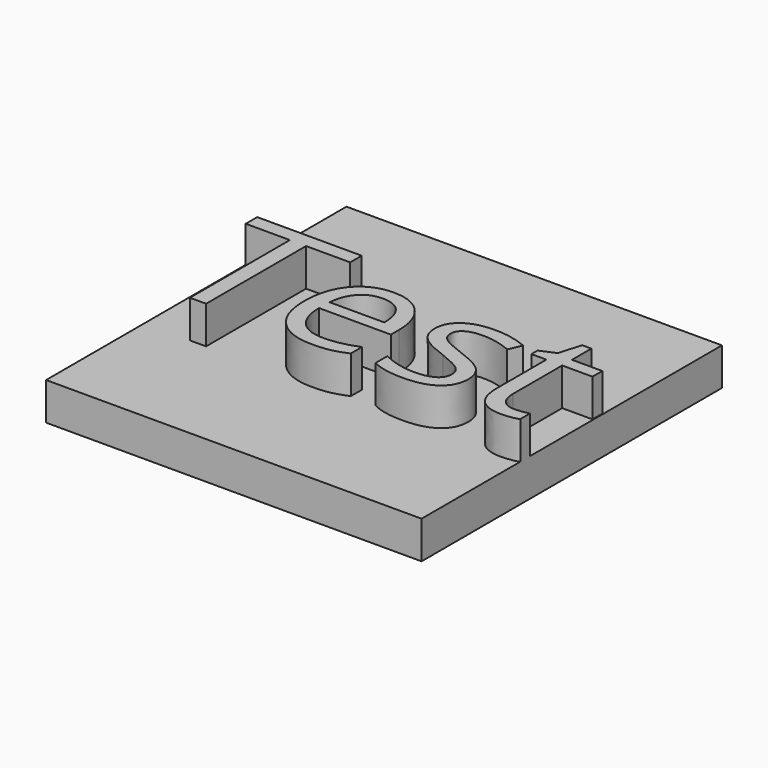
from build123d import *

# Parameters (mm, degrees)
F1_W         = 25.4
F1_H         = 25.4
F2_DEPTH     = 2.54
F0_TEXT_SIZE = 13.2055239643
F3_DEPTH     = 2.54


# Not quite as in the source:
# - Text() gives the source's letters only with a copy of the font that has no kerning and outlines rounded to 1/6400 em; it was checked with that copy


with BuildPart() as f2:
    # F1 (on Top) → F2 (new body)
    with BuildSketch(Plane.XY):
        Rectangle(F1_W, F1_H)
    extrude(amount=F2_DEPTH)

    # F0 (on face) → F3 (join)
    with BuildSketch(Plane.XY.offset(2.54)):
        with Locations((-12.7, -4.4160220119)):
            Text('Test', F0_TEXT_SIZE, font='Open Sans', text_align=(TextAlign.LEFT, TextAlign.BOTTOM))
    extrude(amount=F3_DEPTH)


solid = f2.part
